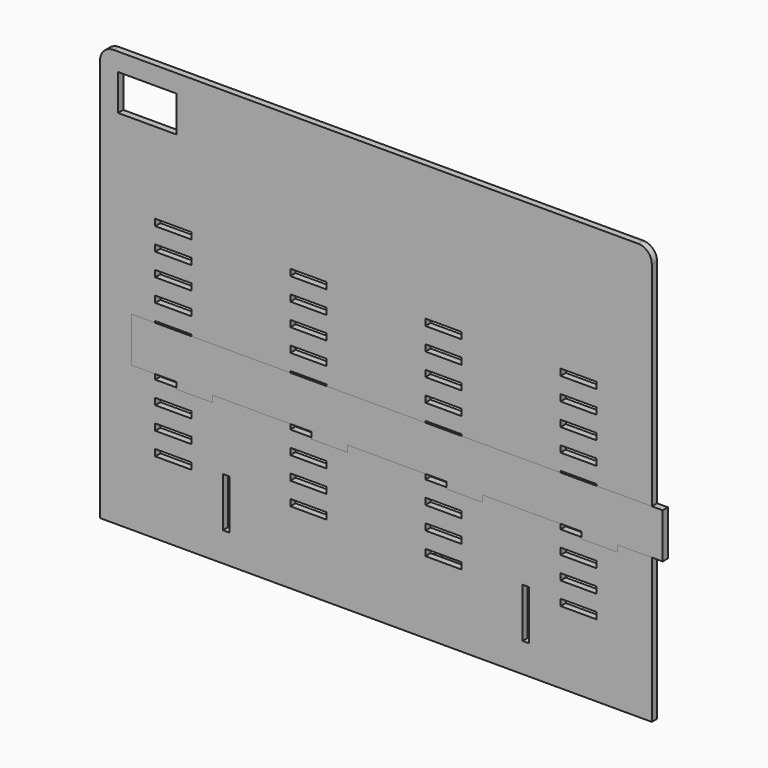
from build123d import *

# Parameters (mm, degrees)
F0_W     = 16
F0_H     = 2.9
F0_W_2   = 2.9
F0_H_2   = 22
F0_W_3   = 26
F0_H_3   = 16
F1_DEPTH = 2.9
F3_DEPTH = 1.45
F5_DEPTH = 2.9


# Not quite as in the source:
# - a feature names something its author has since deleted; it is built from what else it names


with BuildPart() as f1:
    # F0 (on Front) → F1 (new body)
    with BuildSketch(Plane.XZ):
        with BuildLine():
            Line((116.5, 185), (-116.5, 185))
            ThreePointArc((-116.5, 185), (-120.7426406871, 183.2426406871), (-122.5, 179))
            Line((-122.5, 179), (-122.5, 0))
            Line((-122.5, 0), (122.5, 0))
            Line((122.5, 0), (122.5, 179))
            ThreePointArc((122.5, 179), (120.7426406871, 183.2426406871), (116.5, 185))
        make_face()
        with Locations((-90, 33.55)):
            Rectangle(F0_W, F0_H, mode=Mode.SUBTRACT)
        with Locations((-66.55, 24)):
            Rectangle(F0_W_2, F0_H_2, mode=Mode.SUBTRACT)
        with Locations((-90, 43.55)):
            Rectangle(F0_W, F0_H, mode=Mode.SUBTRACT)
        with Locations((-30, 33.55)):
            Rectangle(F0_W, F0_H, mode=Mode.SUBTRACT)
        with Locations((-30, 43.55)):
            Rectangle(F0_W, F0_H, mode=Mode.SUBTRACT)
        with Locations((-90, 53.55)):
            Rectangle(F0_W, F0_H, mode=Mode.SUBTRACT)
        with Locations((-90, 63.55)):
            Rectangle(F0_W, F0_H, mode=Mode.SUBTRACT)
        with Locations((-90, 73.55)):
            Rectangle(F0_W, F0_H, mode=Mode.SUBTRACT)
        with Locations((-90, 83.55)):
            Rectangle(F0_W, F0_H, mode=Mode.SUBTRACT)
        with Locations((-30, 53.55)):
            Rectangle(F0_W, F0_H, mode=Mode.SUBTRACT)
        with Locations((-30, 63.55)):
            Rectangle(F0_W, F0_H, mode=Mode.SUBTRACT)
        with Locations((-30, 73.55)):
            Rectangle(F0_W, F0_H, mode=Mode.SUBTRACT)
        with Locations((-30, 83.55)):
            Rectangle(F0_W, F0_H, mode=Mode.SUBTRACT)
        with Locations((30, 33.55)):
            Rectangle(F0_W, F0_H, mode=Mode.SUBTRACT)
        with Locations((30, 43.55)):
            Rectangle(F0_W, F0_H, mode=Mode.SUBTRACT)
        with Locations((66.55, 24)):
            Rectangle(F0_W_2, F0_H_2, mode=Mode.SUBTRACT)
        with Locations((90, 33.55)):
            Rectangle(F0_W, F0_H, mode=Mode.SUBTRACT)
        with Locations((90, 43.55)):
            Rectangle(F0_W, F0_H, mode=Mode.SUBTRACT)
        with Locations((30, 53.55)):
            Rectangle(F0_W, F0_H, mode=Mode.SUBTRACT)
        with Locations((30, 63.55)):
            Rectangle(F0_W, F0_H, mode=Mode.SUBTRACT)
        with Locations((30, 73.55)):
            Rectangle(F0_W, F0_H, mode=Mode.SUBTRACT)
        with Locations((30, 83.55)):
            Rectangle(F0_W, F0_H, mode=Mode.SUBTRACT)
        with Locations((90, 53.55)):
            Rectangle(F0_W, F0_H, mode=Mode.SUBTRACT)
        with Locations((90, 63.55)):
            Rectangle(F0_W, F0_H, mode=Mode.SUBTRACT)
        with Locations((90, 73.55)):
            Rectangle(F0_W, F0_H, mode=Mode.SUBTRACT)
        with Locations((90, 83.55)):
            Rectangle(F0_W, F0_H, mode=Mode.SUBTRACT)
        with Locations((-90, 93.55)):
            Rectangle(F0_W, F0_H, mode=Mode.SUBTRACT)
        with Locations((-90, 103.55)):
            Rectangle(F0_W, F0_H, mode=Mode.SUBTRACT)
        with Locations((-90, 113.55)):
            Rectangle(F0_W, F0_H, mode=Mode.SUBTRACT)
        with Locations((-90, 123.55)):
            Rectangle(F0_W, F0_H, mode=Mode.SUBTRACT)
        with Locations((-30, 93.55)):
            Rectangle(F0_W, F0_H, mode=Mode.SUBTRACT)
        with Locations((-30, 103.55)):
            Rectangle(F0_W, F0_H, mode=Mode.SUBTRACT)
        with Locations((-30, 113.55)):
            Rectangle(F0_W, F0_H, mode=Mode.SUBTRACT)
        with Locations((-30, 123.55)):
            Rectangle(F0_W, F0_H, mode=Mode.SUBTRACT)
        with Locations((-101.5, 169)):
            Rectangle(F0_W_3, F0_H_3, mode=Mode.SUBTRACT)
        with Locations((30, 93.55)):
            Rectangle(F0_W, F0_H, mode=Mode.SUBTRACT)
        with Locations((30, 103.55)):
            Rectangle(F0_W, F0_H, mode=Mode.SUBTRACT)
        with Locations((30, 113.55)):
            Rectangle(F0_W, F0_H, mode=Mode.SUBTRACT)
        with Locations((30, 123.55)):
            Rectangle(F0_W, F0_H, mode=Mode.SUBTRACT)
        with Locations((90, 93.55)):
            Rectangle(F0_W, F0_H, mode=Mode.SUBTRACT)
        with Locations((90, 103.55)):
            Rectangle(F0_W, F0_H, mode=Mode.SUBTRACT)
        with Locations((90, 113.55)):
            Rectangle(F0_W, F0_H, mode=Mode.SUBTRACT)
        with Locations((90, 123.55)):
            Rectangle(F0_W, F0_H, mode=Mode.SUBTRACT)
    extrude(amount=F1_DEPTH)


with BuildPart() as f3:
    # F2 (on Right) → F3 (new body, symmetric)
    with BuildSketch(Plane.YZ):
        Polygon((6.5, 11.2583302492), (0, 0), (125, 0), (18.2493059725, 13.1073370922), (27.5, 47.6313972081), (17.5, 30.3108891325), (14.988526329, 31.7608891325), (3.988526329, 12.7083302492), align=None)
    extrude(amount=F3_DEPTH, both=True)


with BuildPart() as f5:
    # F4 (on Front) → F5 (new body)
    with BuildSketch(Plane.XZ):
        Polygon((-108.6425621135, 84.2970302286), (-108.6425621135, 64.2970302286), (-88.6425621135, 64.2970302286), (-88.6425621135, 61.3970302286), (-72.6425621135, 61.3970302286), (-72.6425621135, 64.2970302286), (-28.6425621135, 64.2970302286), (-28.6425621135, 61.3970302286), (-12.6425621135, 61.3970302286), (-12.6425621135, 64.2970302286), (31.3574378865, 64.2970302286), (31.3574378865, 61.3970302286), (47.3574378865, 61.3970302286), (47.3574378865, 64.2970302286), (91.3574378865, 64.2970302286), (91.3574378865, 61.3970302286), (107.3574378865, 61.3970302286), (107.3574378865, 64.2970302286), (127.3574378865, 64.2970302286), (127.3574378865, 84.2970302286), align=None)
    extrude(amount=F5_DEPTH)


solid = Compound([f1.part, f3.part, f5.part])
